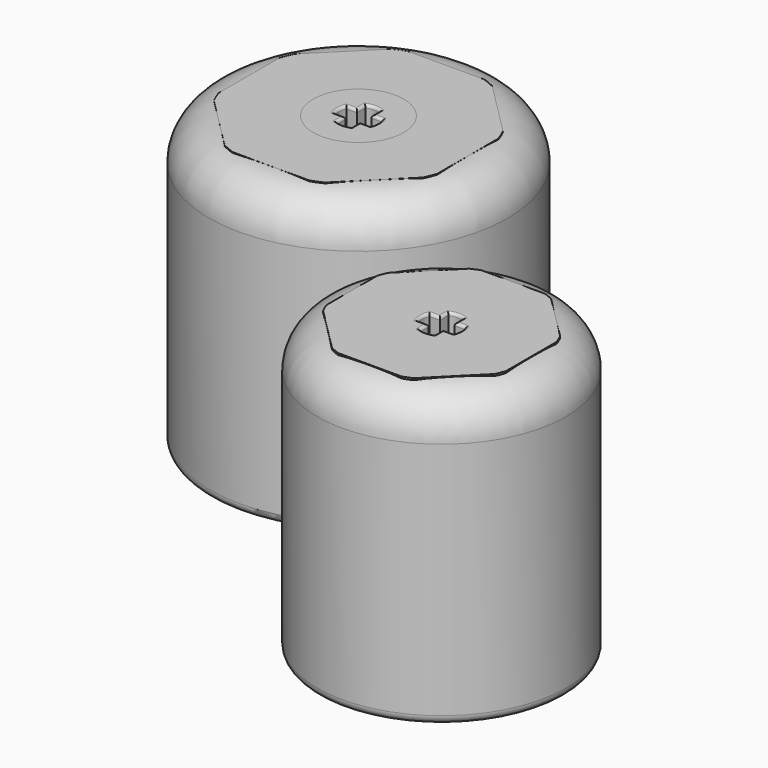
from build123d import *

# Parameters (mm, degrees)
F1_START = 25.4
F1_DEPTH = 2.54
F2_START = 25.4
F0_R     = 6.35
F2_DEPTH = 15.24
F3_START = 25.4
F3_DEPTH = 15.24
F0_R_2   = 17.4625
F4_DEPTH = 40.64
F0_R_3   = 20.955
F5_R     = 0.381
F5_2_R   = 0.381
F7_R     = 1.27
F7_2_R   = 1.27


# Not quite as in the source:
# - a fillet or chamfer that OpenCascade refuses, or shapes differently, is made with other operations: its cross-section is extruded or revolved along the edge and cut away or added


with BuildPart() as f1:
    # F0 (on Top) → F1 (new body)
    with BuildSketch(Plane.XY.offset(F1_START)):
        with BuildLine():
            Line((2.5029669894, 1.0125), (1.0125, 1.0125))
            Line((1.0125, 1.0125), (1.0125, 2.5029669894))
            ThreePointArc((1.0125, 2.5029669894), (0, 2.7), (-1.0125, 2.5029669894))
            Line((-1.0125, 2.5029669894), (-1.0125, 1.0125))
            Line((-1.0125, 1.0125), (-2.5029669894, 1.0125))
            ThreePointArc((-2.5029669894, 1.0125), (-2.7, 0), (-2.5029669894, -1.0125))
            Line((-2.5029669894, -1.0125), (-1.0125, -1.0125))
            Line((-1.0125, -1.0125), (-1.0125, -2.5029669894))
            ThreePointArc((-1.0125, -2.5029669894), (0, -2.7), (1.0125, -2.5029669894))
            Line((1.0125, -2.5029669894), (1.0125, -1.0125))
            Line((1.0125, -1.0125), (2.5029669894, -1.0125))
            ThreePointArc((2.5029669894, -1.0125), (2.7, 0), (2.5029669894, 1.0125))
        make_face()
    extrude(amount=F1_DEPTH)

    # F0 (on Top) → F2 (join)
    with BuildSketch(Plane.XY.offset(F2_START)):
        Circle(F0_R)
        with BuildLine():
            Line((1.0125, 2.5029669894), (1.0125, 1.0125))
            Line((1.0125, 1.0125), (2.5029669894, 1.0125))
            ThreePointArc((2.5029669894, 1.0125), (2.7, 0), (2.5029669894, -1.0125))
            Line((2.5029669894, -1.0125), (1.0125, -1.0125))
            Line((1.0125, -1.0125), (1.0125, -2.5029669894))
            ThreePointArc((1.0125, -2.5029669894), (0, -2.7), (-1.0125, -2.5029669894))
            Line((-1.0125, -2.5029669894), (-1.0125, -1.0125))
            Line((-1.0125, -1.0125), (-2.5029669894, -1.0125))
            ThreePointArc((-2.5029669894, -1.0125), (-2.7, 0), (-2.5029669894, 1.0125))
            Line((-2.5029669894, 1.0125), (-1.0125, 1.0125))
            Line((-1.0125, 1.0125), (-1.0125, 2.5029669894))
            ThreePointArc((-1.0125, 2.5029669894), (0, 2.7), (1.0125, 2.5029669894))
        make_face(mode=Mode.SUBTRACT)
    extrude(amount=F2_DEPTH)

    # F0 (on Top) → F3 (join)
    with BuildSketch(Plane.XY.offset(F3_START)):
        with BuildLine():
            Line((-5.7486470731, 12.0322600466), (-12.0322600466, 5.7486470731))
            ThreePointArc((-12.0322600466, 5.7486470731), (-12.319933566, 5.1030835706), (-12.573, 4.4431853439))
            Line((-12.573, 4.4431853439), (-12.573, -4.4431853439))
            ThreePointArc((-12.573, -4.4431853439), (-12.319933566, -5.1030835706), (-12.0322600466, -5.7486470731))
            Line((-12.0322600466, -5.7486470731), (-5.7486470731, -12.0322600466))
            ThreePointArc((-5.7486470731, -12.0322600466), (-5.1030835706, -12.319933566), (-4.4431853439, -12.573))
            Line((-4.4431853439, -12.573), (4.4431853439, -12.573))
            ThreePointArc((4.4431853439, -12.573), (5.1030835706, -12.319933566), (5.7486470731, -12.0322600466))
            Line((5.7486470731, -12.0322600466), (12.0322600466, -5.7486470731))
            ThreePointArc((12.0322600466, -5.7486470731), (12.319933566, -5.1030835706), (12.573, -4.4431853439))
            Line((12.573, -4.4431853439), (12.573, 4.4431853439))
            ThreePointArc((12.573, 4.4431853439), (12.319933566, 5.1030835706), (12.0322600466, 5.7486470731))
            Line((12.0322600466, 5.7486470731), (5.7486470731, 12.0322600466))
            ThreePointArc((5.7486470731, 12.0322600466), (5.1030835706, 12.319933566), (4.4431853439, 12.573))
            Line((4.4431853439, 12.573), (-4.4431853439, 12.573))
            ThreePointArc((-4.4431853439, 12.573), (-5.1030835706, 12.319933566), (-5.7486470731, 12.0322600466))
        make_face()
        Circle(F0_R, mode=Mode.SUBTRACT)
    extrude(amount=F3_DEPTH)

    # F5
    f5_edges = [f1.edges().sort_by_distance(p)[0] for p in [
        (1.0125, -1.757733, 40.64),
        (2.7, 0, 40.64),
        (1.757733, 1.0125, 40.64),
        (1.757733, -1.0125, 40.64),
        (0, -2.7, 40.64),
        (-1.0125, -1.757733, 40.64),
        (-2.7, 0, 40.64),
        (-1.757733, -1.0125, 40.64),
        (-1.757733, 1.0125, 40.64),
        (-1.0125, 1.757733, 40.64),
        (0, 2.7, 40.64),
        (1.0125, 1.757733, 40.64),
    ]]
    fillet(f5_edges, radius=F5_R)


with BuildPart() as f1b:
    # F0 (on Top) → F1, piece 2 (new body)
    with BuildSketch(Plane.XY.offset(F1_START)):
        with BuildLine():
            Line((-40.3893615403, 31.7689274535), (-38.8988945509, 31.7689274535))
            Line((-38.8988945509, 31.7689274535), (-38.8988945509, 30.2784604641))
            ThreePointArc((-38.8988945509, 30.2784604641), (-37.8863945509, 30.0814274535), (-36.8738945509, 30.2784604641))
            Line((-36.8738945509, 30.2784604641), (-36.8738945509, 31.7689274535))
            Line((-36.8738945509, 31.7689274535), (-35.3834275615, 31.7689274535))
            ThreePointArc((-35.3834275615, 31.7689274535), (-35.1863945509, 32.7814274535), (-35.3834275615, 33.7939274535))
            Line((-35.3834275615, 33.7939274535), (-36.8738945509, 33.7939274535))
            Line((-36.8738945509, 33.7939274535), (-36.8738945509, 35.2843944429))
            ThreePointArc((-36.8738945509, 35.2843944429), (-37.8863945509, 35.4814274535), (-38.8988945509, 35.2843944429))
            Line((-38.8988945509, 35.2843944429), (-38.8988945509, 33.7939274535))
            Line((-38.8988945509, 33.7939274535), (-40.3893615403, 33.7939274535))
            ThreePointArc((-40.3893615403, 33.7939274535), (-40.5863945509, 32.7814274535), (-40.3893615403, 31.7689274535))
        make_face()
    extrude(amount=F1_DEPTH)


with BuildPart() as f2:
    # F0 (on Top) → F2, piece 2 (new body)
    with BuildSketch(Plane.XY.offset(F2_START)):
        with Locations((-37.8863945509, 32.7814274535)):
            Circle(F0_R)
        with BuildLine():
            Line((-38.8988945509, 30.2784604641), (-38.8988945509, 31.7689274535))
            Line((-38.8988945509, 31.7689274535), (-40.3893615403, 31.7689274535))
            ThreePointArc((-40.3893615403, 31.7689274535), (-40.5863945509, 32.7814274535), (-40.3893615403, 33.7939274535))
            Line((-40.3893615403, 33.7939274535), (-38.8988945509, 33.7939274535))
            Line((-38.8988945509, 33.7939274535), (-38.8988945509, 35.2843944429))
            ThreePointArc((-38.8988945509, 35.2843944429), (-37.8863945509, 35.4814274535), (-36.8738945509, 35.2843944429))
            Line((-36.8738945509, 35.2843944429), (-36.8738945509, 33.7939274535))
            Line((-36.8738945509, 33.7939274535), (-35.3834275615, 33.7939274535))
            ThreePointArc((-35.3834275615, 33.7939274535), (-35.1863945509, 32.7814274535), (-35.3834275615, 31.7689274535))
            Line((-35.3834275615, 31.7689274535), (-36.8738945509, 31.7689274535))
            Line((-36.8738945509, 31.7689274535), (-36.8738945509, 30.2784604641))
            ThreePointArc((-36.8738945509, 30.2784604641), (-37.8863945509, 30.0814274535), (-38.8988945509, 30.2784604641))
        make_face(mode=Mode.SUBTRACT)
    extrude(amount=F2_DEPTH)

    # F5#2
    f5_2_edges = [f2.edges().sort_by_distance(p)[0] for p in [
        (-36.128661, 33.793927, 40.64),
        (-35.186395, 32.781427, 40.64),
        (-36.873895, 31.023694, 40.64),
        (-36.873895, 34.539161, 40.64),
        (-37.886395, 35.481427, 40.64),
        (-36.128661, 31.768927, 40.64),
        (-39.644128, 33.793927, 40.64),
        (-38.898895, 34.539161, 40.64),
        (-39.644128, 31.768927, 40.64),
        (-40.586395, 32.781427, 40.64),
        (-38.898895, 31.023694, 40.64),
        (-37.886395, 30.081427, 40.64),
    ]]
    fillet(f5_2_edges, radius=F5_2_R)


with BuildPart() as f3:
    # F0 (on Top) → F3, piece 2 (new body)
    with BuildSketch(Plane.XY.offset(F3_START)):
        with BuildLine():
            Line((-22.5447945509, 27.4062209049), (-22.5447945509, 38.1566340021))
            ThreePointArc((-22.5447945509, 38.1566340021), (-22.8678088704, 39.00232933), (-23.2374001559, 39.8287318469))
            Line((-23.2374001559, 39.8287318469), (-30.8390901575, 47.4304218485))
            ThreePointArc((-30.8390901575, 47.4304218485), (-31.6654926744, 47.800013134), (-32.5111880023, 48.1230274535))
            Line((-32.5111880023, 48.1230274535), (-43.2616010995, 48.1230274535))
            ThreePointArc((-43.2616010995, 48.1230274535), (-44.1072964275, 47.800013134), (-44.9336989444, 47.4304218485))
            Line((-44.9336989444, 47.4304218485), (-52.535388946, 39.8287318469))
            ThreePointArc((-52.535388946, 39.8287318469), (-52.9049802314, 39.00232933), (-53.2279945509, 38.1566340021))
            Line((-53.2279945509, 38.1566340021), (-53.2279945509, 27.4062209049))
            ThreePointArc((-53.2279945509, 27.4062209049), (-52.9049802314, 26.5605255769), (-52.535388946, 25.73412306))
            Line((-52.535388946, 25.73412306), (-44.9336989444, 18.1324330584))
            ThreePointArc((-44.9336989444, 18.1324330584), (-44.1072964275, 17.762841773), (-43.2616010995, 17.4398274535))
            Line((-43.2616010995, 17.4398274535), (-32.5111880023, 17.4398274535))
            ThreePointArc((-32.5111880023, 17.4398274535), (-31.6654926744, 17.762841773), (-30.8390901575, 18.1324330584))
            Line((-30.8390901575, 18.1324330584), (-23.2374001559, 25.73412306))
            ThreePointArc((-23.2374001559, 25.73412306), (-22.8678088704, 26.5605255769), (-22.5447945509, 27.4062209049))
        make_face()
        with Locations((-37.8863945509, 32.7814274535)):
            Circle(F0_R, mode=Mode.SUBTRACT)
    extrude(amount=F3_DEPTH)


with BuildPart() as f4:
    # F0 (on Top) → F4 (new body)
    with BuildSketch(Plane.XY):
        Circle(F0_R_2)
        with BuildLine():
            ThreePointArc((-12.573, 4.4431853439), (-12.319933566, 5.1030835706), (-12.0322600466, 5.7486470731))
            Line((-12.0322600466, 5.7486470731), (-5.7486470731, 12.0322600466))
            ThreePointArc((-5.7486470731, 12.0322600466), (-5.1030835706, 12.319933566), (-4.4431853439, 12.573))
            Line((-4.4431853439, 12.573), (4.4431853439, 12.573))
            ThreePointArc((4.4431853439, 12.573), (5.1030835706, 12.319933566), (5.7486470731, 12.0322600466))
            Line((5.7486470731, 12.0322600466), (12.0322600466, 5.7486470731))
            ThreePointArc((12.0322600466, 5.7486470731), (12.319933566, 5.1030835706), (12.573, 4.4431853439))
            Line((12.573, 4.4431853439), (12.573, -4.4431853439))
            ThreePointArc((12.573, -4.4431853439), (12.319933566, -5.1030835706), (12.0322600466, -5.7486470731))
            Line((12.0322600466, -5.7486470731), (5.7486470731, -12.0322600466))
            ThreePointArc((5.7486470731, -12.0322600466), (5.1030835706, -12.319933566), (4.4431853439, -12.573))
            Line((4.4431853439, -12.573), (-4.4431853439, -12.573))
            ThreePointArc((-4.4431853439, -12.573), (-5.1030835706, -12.319933566), (-5.7486470731, -12.0322600466))
            Line((-5.7486470731, -12.0322600466), (-12.0322600466, -5.7486470731))
            ThreePointArc((-12.0322600466, -5.7486470731), (-12.319933566, -5.1030835706), (-12.573, -4.4431853439))
            Line((-12.573, -4.4431853439), (-12.573, 4.4431853439))
        make_face(mode=Mode.SUBTRACT)
    extrude(amount=F4_DEPTH)

    # F6: fillet of radius 5.842 on 1 edges, made by hand

    # F6_s1 → F6_t2 (revolve, cut)
    with BuildSketch(Plane.XZ):
        with BuildLine():
            ThreePointArc((17.4625, 34.798), (15.7514178157, 38.9289178157), (11.6205, 40.64))
            Line((11.6205, 40.64), (17.4625, 40.64))
            Line((17.4625, 40.64), (17.4625, 34.798))
        make_face()
    revolve(axis=Axis((0, 0, 40.64), (0, 0, 1)), mode=Mode.SUBTRACT)

    # F7
    f7_edges = [f4.edges().sort_by_distance(p)[0] for p in [
        (-17.4625, 0, 0),
        (-8.890454, -8.890454, 0),
        (-12.573, 0, 0),
        (-12.319934, -5.103084, 0),
        (-5.103084, -12.319934, 0),
        (0, -12.573, 0),
        (5.103084, -12.319934, 0),
        (8.890454, -8.890454, 0),
        (-8.890454, 8.890454, 0),
        (-12.319934, 5.103084, 0),
        (-5.103084, 12.319934, 0),
        (0, 12.573, 0),
        (5.103084, 12.319934, 0),
        (8.890454, 8.890454, 0),
        (12.319934, 5.103084, 0),
        (12.573, 0, 0),
        (12.319934, -5.103084, 0),
    ]]
    fillet(f7_edges, radius=F7_R)


with BuildPart() as f4b:
    # F0 (on Top) → F4, piece 2 (new body)
    with BuildSketch(Plane.XY):
        with Locations((-37.8863945509, 32.7814274535)):
            Circle(F0_R_3)
        with BuildLine():
            ThreePointArc((-23.2374001559, 39.8287318469), (-22.8678088704, 39.00232933), (-22.5447945509, 38.1566340021))
            Line((-22.5447945509, 38.1566340021), (-22.5447945509, 27.4062209049))
            ThreePointArc((-22.5447945509, 27.4062209049), (-22.8678088704, 26.5605255769), (-23.2374001559, 25.73412306))
            Line((-23.2374001559, 25.73412306), (-30.8390901575, 18.1324330584))
            ThreePointArc((-30.8390901575, 18.1324330584), (-31.6654926744, 17.762841773), (-32.5111880023, 17.4398274535))
            Line((-32.5111880023, 17.4398274535), (-43.2616010995, 17.4398274535))
            ThreePointArc((-43.2616010995, 17.4398274535), (-44.1072964275, 17.762841773), (-44.9336989444, 18.1324330584))
            Line((-44.9336989444, 18.1324330584), (-52.535388946, 25.73412306))
            ThreePointArc((-52.535388946, 25.73412306), (-52.9049802314, 26.5605255769), (-53.2279945509, 27.4062209049))
            Line((-53.2279945509, 27.4062209049), (-53.2279945509, 38.1566340021))
            ThreePointArc((-53.2279945509, 38.1566340021), (-52.9049802314, 39.00232933), (-52.535388946, 39.8287318469))
            Line((-52.535388946, 39.8287318469), (-44.9336989444, 47.4304218485))
            ThreePointArc((-44.9336989444, 47.4304218485), (-44.1072964275, 47.800013134), (-43.2616010995, 48.1230274535))
            Line((-43.2616010995, 48.1230274535), (-32.5111880023, 48.1230274535))
            ThreePointArc((-32.5111880023, 48.1230274535), (-31.6654926744, 47.800013134), (-30.8390901575, 47.4304218485))
            Line((-30.8390901575, 47.4304218485), (-23.2374001559, 39.8287318469))
        make_face(mode=Mode.SUBTRACT)
    extrude(amount=F4_DEPTH)

    # F6#2: fillet of radius 5.842 on 1 edges, made by hand

    # F6_2_s1 → F6_2_t2 (revolve, cut)
    with BuildSketch(Plane.XZ.offset(-32.7814274535)):
        with BuildLine():
            ThreePointArc((-16.9313945509, 34.798), (-18.6424767352, 38.9289178157), (-22.7733945509, 40.64))
            Line((-22.7733945509, 40.64), (-16.9313945509, 40.64))
            Line((-16.9313945509, 40.64), (-16.9313945509, 34.798))
        make_face()
    revolve(axis=Axis((-37.8863945509, 32.7814274535, 40.64), (0, 0, 1)), mode=Mode.SUBTRACT)

    # F7#2
    f7_2_edges = [f4b.edges().sort_by_distance(p)[0] for p in [
        (-58.841395, 32.781427, 0),
        (-37.886395, 17.439827, 0),
        (-48.734544, 21.933278, 0),
        (-44.107296, 17.762842, 0),
        (-31.665493, 17.762842, 0),
        (-27.038245, 21.933278, 0),
        (-22.867809, 26.560526, 0),
        (-22.544795, 32.781427, 0),
        (-22.867809, 39.002329, 0),
        (-27.038245, 43.629577, 0),
        (-52.90498, 26.560526, 0),
        (-53.227995, 32.781427, 0),
        (-52.90498, 39.002329, 0),
        (-48.734544, 43.629577, 0),
        (-44.107296, 47.800013, 0),
        (-37.886395, 48.123027, 0),
        (-31.665493, 47.800013, 0),
    ]]
    fillet(f7_2_edges, radius=F7_2_R)


solid = Compound([f1.part, f1b.part, f2.part, f3.part, f4.part, f4b.part])
